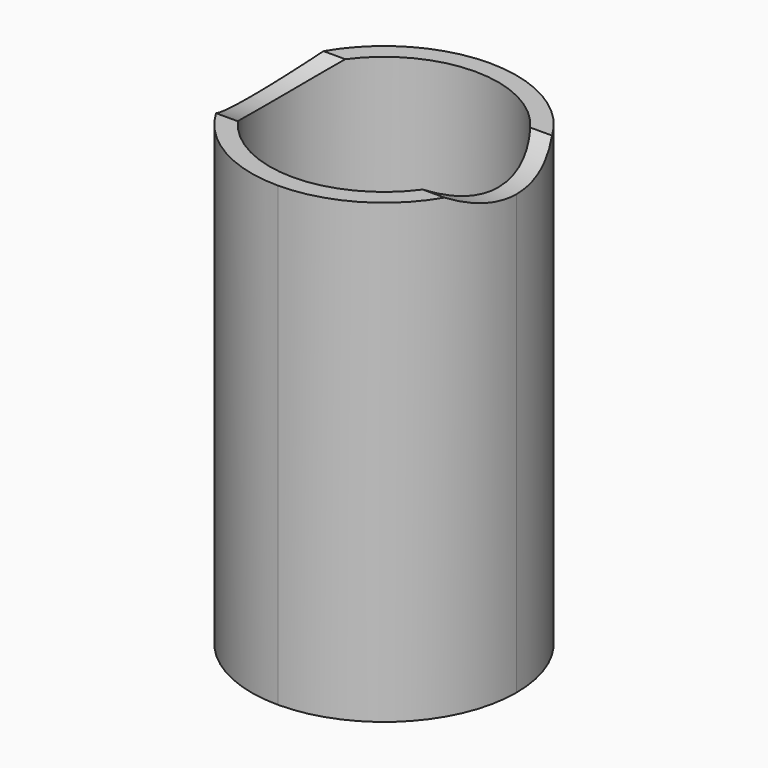
from build123d import *

# Parameters (mm, degrees)
F0_W     = 3.683
F0_H     = 3.683
F0_R     = 1.5875
F1_DEPTH = 6.35
F3_DEPTH = 3.683
F4_R     = 1.84149


# Not quite as in the source:
# - a fillet or chamfer is up to 0.001 mm smaller than in the source, because OpenCascade refuses the exact size


with BuildPart() as f1:
    # F0 (on Top) → F1 (new body)
    with BuildSketch(Plane.XY):
        Rectangle(F0_W, F0_H)
        Circle(F0_R, mode=Mode.SUBTRACT)
    extrude(amount=F1_DEPTH)

    # F2 (on face) → F3 (cut, through all)
    with BuildSketch(Plane.YZ.offset(1.8415)):
        with BuildLine():
            Line((0.933255592, 6.35), (-0.933255592, 6.35))
            ThreePointArc((-0.933255592, 6.35), (0, 6.096), (0.933255592, 6.35))
        make_face()
    extrude(amount=-F3_DEPTH, mode=Mode.SUBTRACT)

    # F4 (radius 1.8415 in the source; OpenCascade refuses exactly that, so slightly less here)
    f4_edges = [f1.edges().sort_by_distance(p)[0] for p in [
        (-1.8415, -1.8415, 3.175),
        (1.8415, -1.8415, 3.175),
        (-1.8415, 1.8415, 3.175),
        (1.8415, 1.8415, 3.175),
    ]]
    fillet(f4_edges, radius=F4_R)


solid = f1.part
